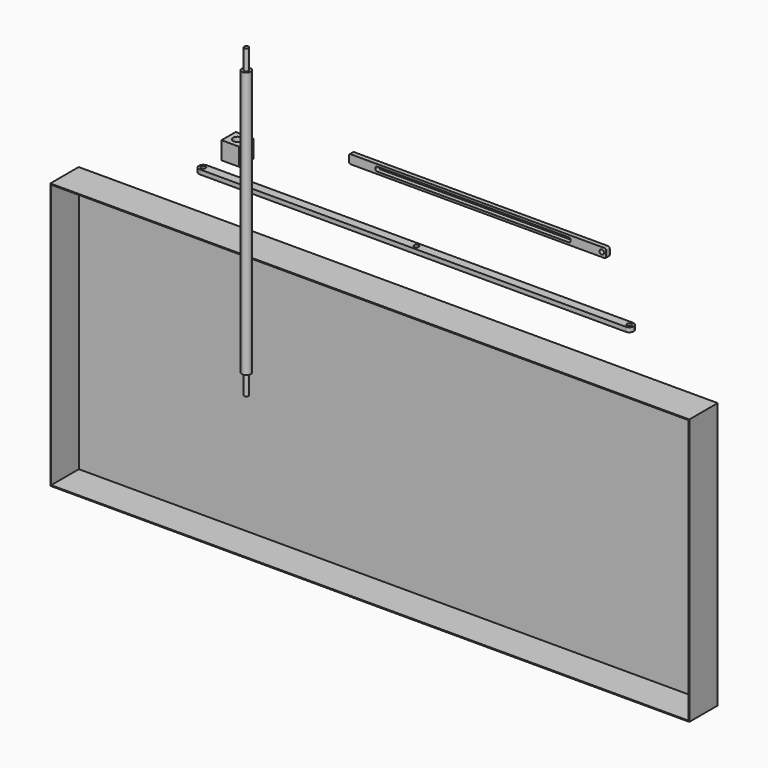
from build123d import *

# Parameters (mm, degrees)
F0_W      = 1244.6
F0_H      = 12.7
F1_DEPTH  = 25.4
F2_R      = 12.69999
F4_D      = 13.49248
F5_R      = 6.35
F6_DEPTH  = 438.15
F5_R_2    = 12.7
F7_DEPTH  = 381
F8_W      = 50.8
F8_H      = 50.8
F9_DEPTH  = 50.8
F11_D     = 25.4
F12_W     = 736.6
F12_H     = 12.7
F13_DEPTH = 25.4
F14_W     = 558.8
F14_H     = 12.7
F15_DEPTH = 236.1610186348
F14_R     = 6.35
F17_R     = 5.08
F18_W     = 1828.8
F18_H     = 762
F19_DEPTH = 101.6
F20_T     = -2.54


# Not quite as in the source:
# - a fillet or chamfer is up to 0.001 mm smaller than in the source, because OpenCascade refuses the exact size


with BuildPart() as f1:
    # F0 (on Front) → F1 (new body)
    with BuildSketch(Plane.XZ):
        with Locations((480.8411406559, 6.35)):
            Rectangle(F0_W, F0_H)
    extrude(amount=F1_DEPTH)

    # F2 (radius 12.7 in the source; OpenCascade refuses exactly that, so slightly less here)
    f2_edges = [f1.edges().sort_by_distance(p)[0] for p in [
        (-141.458859, -25.4, 6.35),
        (1103.141141, -25.4, 6.35),
        (1103.141141, 0, 6.35),
        (-141.458859, 0, 6.35),
    ]]
    fillet(f2_edges, radius=F2_R)

    # F4 (through all)
    with Locations(Plane(origin=(0, 0, 0), x_dir=(1, 0, 0), z_dir=(0, 0, -1))):
        with Locations((480.8411406559, 12.7041507512), (1090.4411406559, 12.7041507512), (-128.7588593441, 12.7041507512)):
            Hole(F4_D / 2)


with BuildPart() as f6:
    # F5 (on Top) → F6 (new body, symmetric)
    with BuildSketch(Plane.XY):
        with Locations((94.2526757717, -137.4980062246)):
            Circle(F5_R)
    extrude(amount=F6_DEPTH, both=True)

    # F5 (on Top) → F7 (join, symmetric)
    with BuildSketch(Plane.XY):
        with Locations((94.2526757717, -137.4980062246)):
            Circle(F5_R_2)
        with Locations((94.2526757717, -137.4980062246)):
            Circle(F5_R, mode=Mode.SUBTRACT)
    extrude(amount=F7_DEPTH, both=True)


with BuildPart() as f9:
    # F8 (on Top) → F9 (new body)
    with BuildSketch(Plane.XY):
        with Locations((-108.0792423666, 83.5509366974)):
            Rectangle(F8_W, F8_H)
    extrude(amount=F9_DEPTH)

    # F11 (through all)
    with Locations(Plane(origin=(0, 0, 0), x_dir=(1, 0, 0), z_dir=(0, 0, -1))):
        with Locations((-108.0792423666, -83.5509366974)):
            Hole(F11_D / 2)


with BuildPart() as f13:
    # F12 (on Top) → F13 (new body)
    with BuildSketch(Plane.XY):
        with Locations((466.9850397587, 229.8100186348)):
            Rectangle(F12_W, F12_H)
    extrude(amount=F13_DEPTH)


with BuildPart() as f15:
    # F14 (on Front) → F15 (new body, through all)
    with BuildSketch(Plane.XZ):
        with Locations((454.2850397587, 12.7)):
            Rectangle(F14_W, F14_H)
    extrude(amount=-F15_DEPTH)


with BuildPart() as f15b:
    # F14 (on Front) → F15, piece 2 (new body, through all)
    with BuildSketch(Plane.XZ):
        with Locations((822.5850397587, 12.7)):
            Circle(F14_R)
    extrude(amount=-F15_DEPTH)


with BuildPart() as f13_1:
    add(f13.part)

    # F16: cut F15, F15b
    add(f15.part, mode=Mode.SUBTRACT)
    add(f15b.part, mode=Mode.SUBTRACT)

    # F17
    f17_edges = [f13_1.edges().sort_by_distance(p)[0] for p in [
        (98.68504, 229.810019, 25.4),
        (835.28504, 229.810019, 25.4),
        (733.68504, 229.810019, 6.35),
        (174.88504, 229.810019, 6.35),
        (174.88504, 229.810019, 19.05),
        (98.68504, 229.810019, 0),
        (835.28504, 229.810019, 0),
        (733.68504, 229.810019, 19.05),
    ]]
    fillet(f17_edges, radius=F17_R)


with BuildPart() as f19:
    # F18 (on Front) → F19 (new body)
    with BuildSketch(Plane.XZ):
        with Locations((418.7591709614, -491.9529797588)):
            Rectangle(F18_W, F18_H)
    extrude(amount=F19_DEPTH)

    # F20
    f20_openings = [f19.faces().sort_by_distance(p)[0] for p in [
        (418.759171, -101.6, -491.95298),
    ]]
    offset(amount=F20_T, openings=f20_openings)


solid = Compound([f1.part, f6.part, f9.part, f13_1.part, f19.part])
